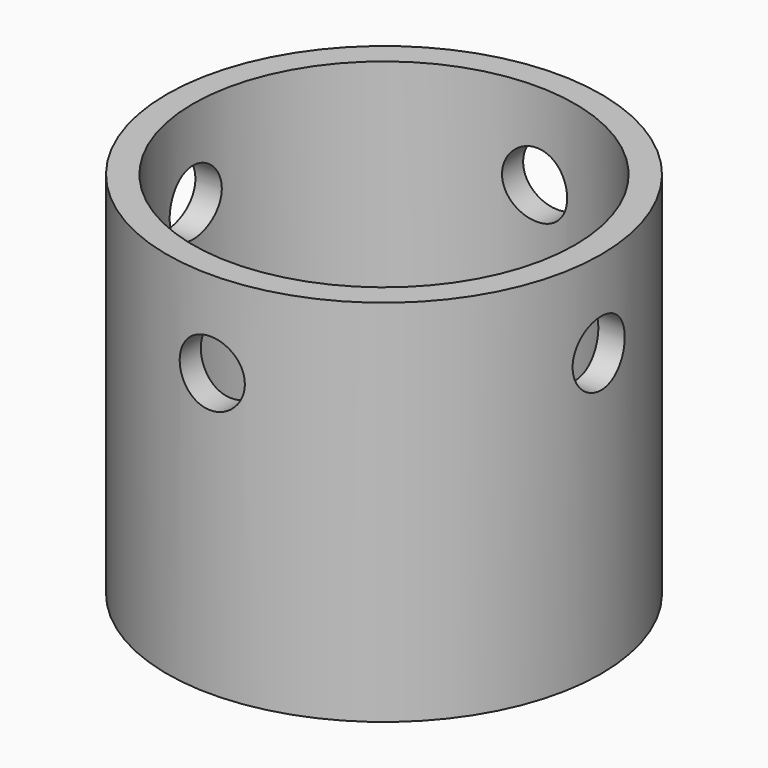
from build123d import *

# Parameters (mm, degrees)
F0_R          = 25.4
F1_DEPTH      = 43.18
F2_R          = 3.81
F3_DEPTH      = 43.181
F4_R          = 3.81
F5_DEPTH      = 25.401
F5_DEPTH_BACK = 25.401
F6_R          = 3.81
F7_DEPTH      = 25.4010001
F7_DEPTH_BACK = 25.4010001
F8_R          = 3.302
F9_DEPTH      = 43.1810001
F10_R         = 22.352
F11_DEPTH     = 40.64


with BuildPart() as f1:
    # F0 (on Top) → F1 (new body)
    with BuildSketch(Plane.XY):
        Circle(F0_R)
    extrude(amount=-F1_DEPTH)

    # F2 (on face) → F3 (cut, through all)
    with BuildSketch(Plane(origin=(0, 0, -43.18), x_dir=(1, 0, 0), z_dir=(0, 0, -1))):
        Circle(F2_R)
    extrude(amount=-F3_DEPTH, mode=Mode.SUBTRACT)

    # F4 (on Right) → F5 (cut, two sides)
    with BuildSketch(Plane.YZ) as f5_sk:
        with Locations((0, -10.16)):
            Circle(F4_R)
    extrude(amount=-F5_DEPTH, mode=Mode.SUBTRACT)
    extrude(f5_sk.sketch, amount=F5_DEPTH_BACK, mode=Mode.SUBTRACT)

    # F6 (on Front) → F7 (cut, two sides)
    with BuildSketch(Plane.XZ) as f7_sk:
        with Locations((0, -10.16)):
            Circle(F6_R)
    extrude(amount=-F7_DEPTH, mode=Mode.SUBTRACT)
    extrude(f7_sk.sketch, amount=F7_DEPTH_BACK, mode=Mode.SUBTRACT)

    # F8 (on face) → F9 (cut, through all)
    with BuildSketch(Plane(origin=(0, 0, -43.18), x_dir=(1, 0, 0), z_dir=(0, 0, -1))):
        with Locations((10.9096324106, 0)):
            Circle(F8_R)
        with Locations((-10.8710342307, 0)):
            Circle(F8_R)
    extrude(amount=-F9_DEPTH, mode=Mode.SUBTRACT)

    # F10 (on face) → F11 (cut)
    with BuildSketch(Plane.XY):
        Circle(F10_R)
    extrude(amount=-F11_DEPTH, mode=Mode.SUBTRACT)


solid = f1.part
